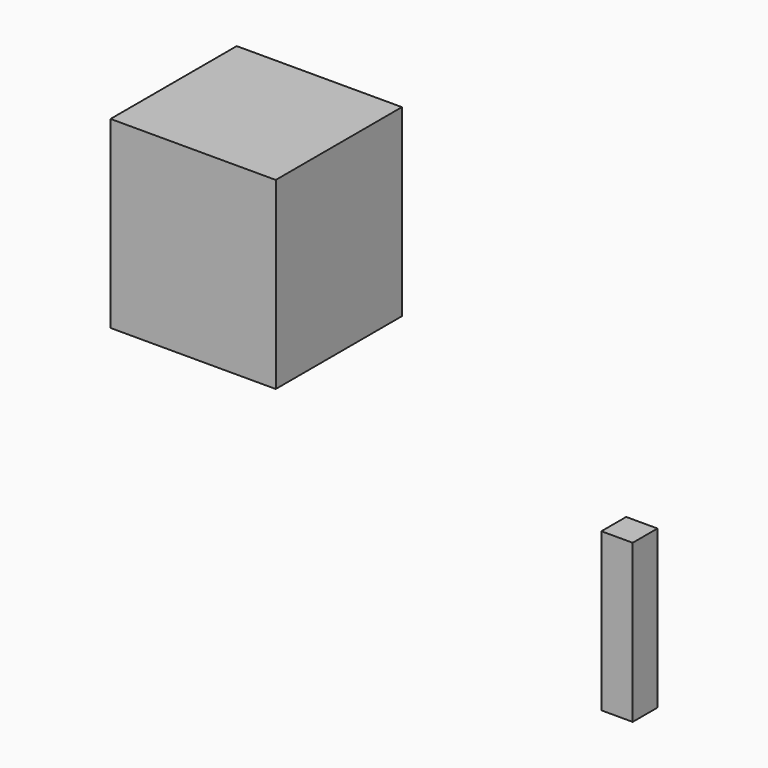
from build123d import *

# Parameters (mm, degrees)
F0_W     = 151.1403471231
F0_H     = 149.6643647552
F1_DEPTH = 762
F6_W     = 798.2519865036
F6_H     = 889.3822431564
F7_DEPTH = 762
F8_W     = 468.693330884
F8_H     = 696.3945627213
F9_DEPTH = 762


# Not quite as in the source:
# - the program builds the solid bodies; features that only make, move or delete a surface that nothing else refers to are left out


with BuildPart() as f1:
    # F0 (on Top) → F1 (new body)
    with BuildSketch(Plane.XY):
        with Locations((-0.0241398811, 0.4020892084)):
            Rectangle(F0_W, F0_H)
    extrude(amount=F1_DEPTH)


with BuildPart() as f7:
    # F6 (on face) → F7 (new body)
    with BuildSketch(Plane.XZ.offset(74.4300931692)):
        with Locations((-1438.5702013969, 1807.9190850258)):
            Rectangle(F6_W, F6_H)
    extrude(amount=F7_DEPTH)

    # F8 (on face) → F9 (cut)
    with BuildSketch(Plane(origin=(-1837.6961946487, 0, 0), x_dir=(0, -1, 0), z_dir=(-1, 0, 0))):
        with Locations((456.2002047896, 1816.4219260216)):
            Rectangle(F8_W, F8_H)
    extrude(amount=-F9_DEPTH, mode=Mode.SUBTRACT)


solid = Compound([f1.part, f7.part])
